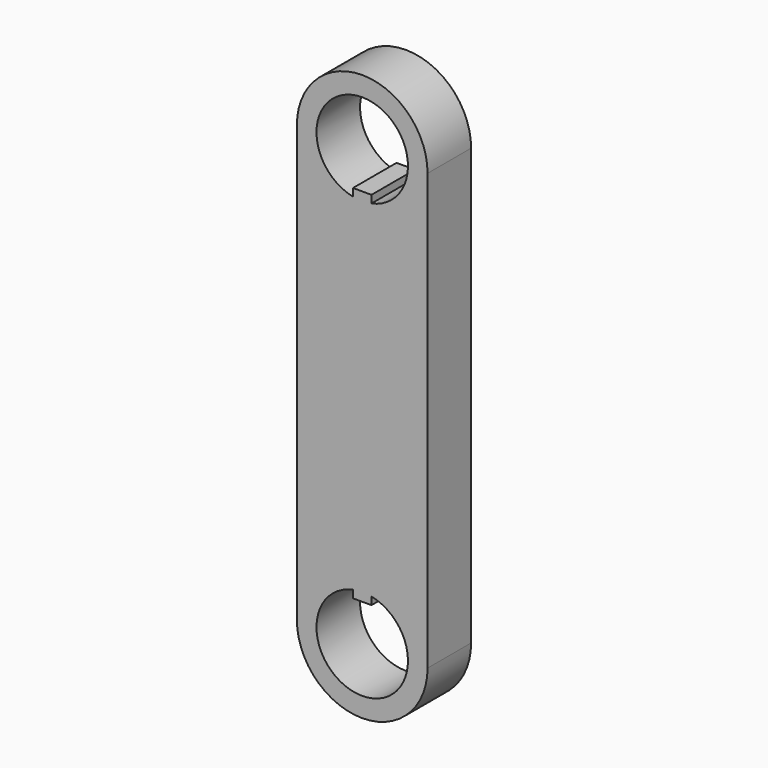
from build123d import *

# Parameters (mm, degrees)
F0_R     = 4.2
F1_DEPTH = 5
F3_DEPTH = 5


# Not quite as in the source:
# - a pattern or mirror of a feature is missing from the dataset's text; its kind, count and spacing are read off the source's solid


with BuildPart() as f1:
    # F0 (on Front) → F1 (new body)
    with BuildSketch(Plane.XZ):
        with BuildLine():
            Line((-6, 40), (-6, 0))
            ThreePointArc((-6, 0), (0, -6), (6, 0))
            Line((6, 0), (6, 40))
            ThreePointArc((6, 40), (0, 46), (-6, 40))
        make_face()
        Circle(F0_R, mode=Mode.SUBTRACT)
        with Locations((0, 40)):
            Circle(F0_R, mode=Mode.SUBTRACT)
    extrude(amount=F1_DEPTH)

    # F2 (on face) → F3 (join, through all)
    with BuildSketch(Plane.XZ.offset(5)):
        Polygon((-0.85, 36.5869111364), (-0.85, 35.8869111364), (0, 14.8420017213), (0.85, 35.8869111364), (0.85, 36.5869111364), align=None)
    f3 = extrude(amount=-F3_DEPTH)

    # F3_copies: F3 across plane
    add(f3.mirror(Plane(origin=(0, 0, 20), x_dir=(-1, 0, 0), z_dir=(0, 0, -1))))


solid = f1.part
